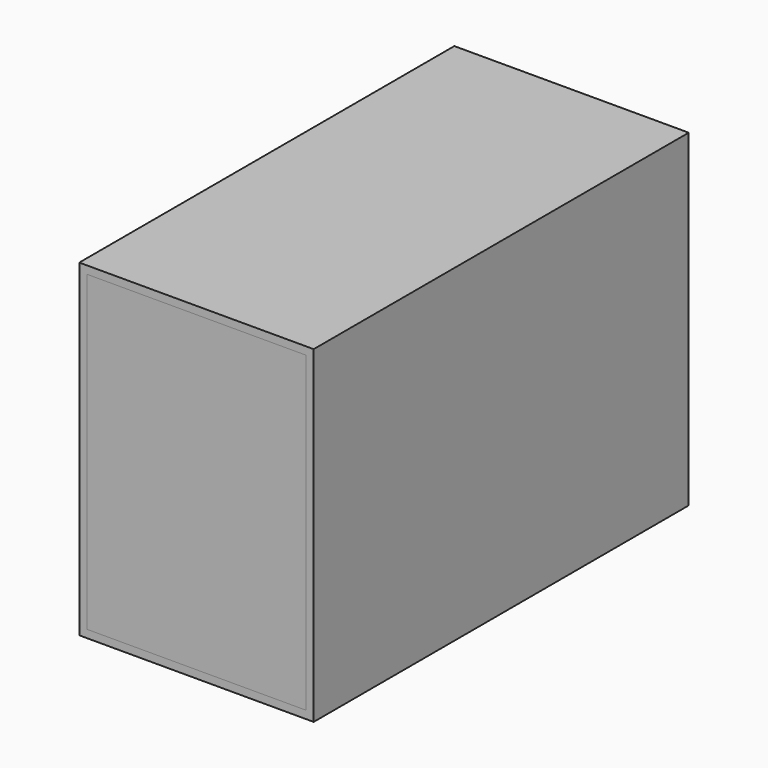
from build123d import *

# Parameters (mm, degrees)
F0_W          = 149.9999934435
F0_H          = 209.9999934435
F0_W_2        = 140
F0_H_2        = 200
F1_DEPTH      = 300
F3_DEPTH      = 70
F3_DEPTH_BACK = 70
F4_DEPTH      = 70
F4_DEPTH_BACK = 70
F5_W          = 140
F5_H          = 200
F6_DEPTH      = 300


with BuildPart() as f1:
    # F0 (on Front) → F1 (new body)
    with BuildSketch(Plane.XZ):
        Rectangle(F0_W, F0_H)
        Rectangle(F0_W_2, F0_H_2, mode=Mode.SUBTRACT)
    extrude(amount=-F1_DEPTH)


with BuildPart() as f3:
    # F2 (on Right) → F3 (new body, two sides)
    with BuildSketch(Plane.YZ) as f3_sk:
        with BuildLine():
            Line((196.2132034356, 29.3933982822), (164.3933982822, 61.2132034356))
            Line((164.3933982822, 61.2132034356), (150, 66.6066017178))
            Line((150, 66.6066017178), (105.2509304011, 63.1825119437))
            ThreePointArc((105.2509304011, 63.1825119437), (99.7778999204, 58.1086464805), (103.4808305396, 51.6289490947))
            Line((103.4808305396, 51.6289490947), (185.6066017178, 18.7867965644))
            Line((185.6066017178, 18.7867965644), (196.2132034356, 29.3933982822))
        make_face()
    extrude(amount=-F3_DEPTH)
    extrude(f3_sk.sketch, amount=F3_DEPTH_BACK)


with BuildPart() as f4:
    # F2 (on Right) → F4 (new body, two sides)
    with BuildSketch(Plane.YZ) as f4_sk:
        with BuildLine():
            Line((185.6066017178, -61.2132034356), (196.2132034356, -50.6066017178))
            Line((196.2132034356, -50.6066017178), (164.3933982822, -18.7867965644))
            Line((164.3933982822, -18.7867965644), (75.424236051, -15.0090028639))
            ThreePointArc((75.424236051, -15.0090028639), (65.2782747437, -22.6573395378), (70.8268318838, -34.0876106801))
            Line((70.8268318838, -34.0876106801), (129.8963013047, -61.2132034356))
            Line((129.8963013047, -61.2132034356), (185.6066017178, -61.2132034356))
        make_face()
    extrude(amount=-F4_DEPTH)
    extrude(f4_sk.sketch, amount=F4_DEPTH_BACK)


with BuildPart() as f6:
    # F5 (on Front) → F6 (new body)
    with BuildSketch(Plane.XZ):
        Rectangle(F5_W, F5_H)
    extrude(amount=-F6_DEPTH)

    # F7: cut F3, F4
    add(f3.part, mode=Mode.SUBTRACT)
    add(f4.part, mode=Mode.SUBTRACT)


solid = Compound([f1.part, f3.part, f4.part, f6.part])
